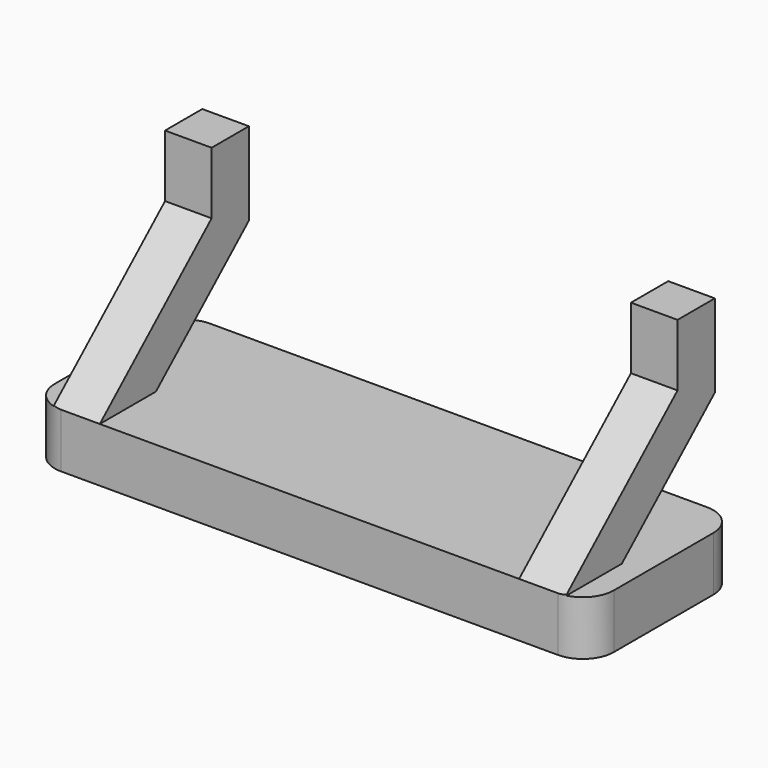
from build123d import *

# Parameters (mm, degrees)
F0_W        = 914.4
F0_H        = 304.8
F1_DEPTH    = 88.9
F2_W        = 76.2
F2_H        = 304.8
F3_DEPTH    = 304.8
F5_DEPTH    = 876.301
F6_T1_DEPTH = 342.9


# Not quite as in the source:
# - a fillet or chamfer that OpenCascade refuses, or shapes differently, is made with other operations: its cross-section is extruded or revolved along the edge and cut away or added


with BuildPart() as f1:
    # F0 (on Top) → F1 (new body)
    with BuildSketch(Plane.XY):
        Rectangle(F0_W, F0_H)
    extrude(amount=F1_DEPTH)

    # F2 (on face) → F3 (join)
    with BuildSketch(Plane.XY.offset(88.9)):
        with Locations((-381, 0)):
            Rectangle(F2_W, F2_H)
        with Locations((381, 0)):
            Rectangle(F2_W, F2_H)
    extrude(amount=F3_DEPTH)

    # F4 (on face) → F5 (cut, through all)
    with BuildSketch(Plane.YZ.offset(419.1)):
        Polygon((76.2, 292.1), (76.2, 393.7), (-152.4, 393.7), (-152.4, 88.9), align=None)
        Polygon((152.4, 88.9), (152.4, 257.8811658996), (-37.703811637, 88.9), align=None)
    extrude(amount=-F5_DEPTH, mode=Mode.SUBTRACT)

    # F6: fillet of radius 50.8 on 4 edges, made by hand

    # F6_s2 → F6_t1 (cut)
    with BuildSketch(Plane.XY.offset(-127)):
        with BuildLine():
            ThreePointArc((-457.2, -101.6), (-442.3210244843, -137.5210244843), (-406.4, -152.4))
            Line((-406.4, -152.4), (-457.2, -152.4))
            Line((-457.2, -152.4), (-457.2, -101.6))
        make_face()
        with BuildLine():
            ThreePointArc((457.2, -101.6), (442.3210244843, -137.5210244843), (406.4, -152.4))
            Line((406.4, -152.4), (457.2, -152.4))
            Line((457.2, -152.4), (457.2, -101.6))
        make_face()
        with BuildLine():
            ThreePointArc((457.2, 101.6), (442.3210244843, 137.5210244843), (406.4, 152.4))
            Line((406.4, 152.4), (457.2, 152.4))
            Line((457.2, 152.4), (457.2, 101.6))
        make_face()
        with BuildLine():
            ThreePointArc((-457.2, 101.6), (-442.3210244843, 137.5210244843), (-406.4, 152.4))
            Line((-406.4, 152.4), (-457.2, 152.4))
            Line((-457.2, 152.4), (-457.2, 101.6))
        make_face()
    extrude(amount=F6_T1_DEPTH, mode=Mode.SUBTRACT)


solid = f1.part
